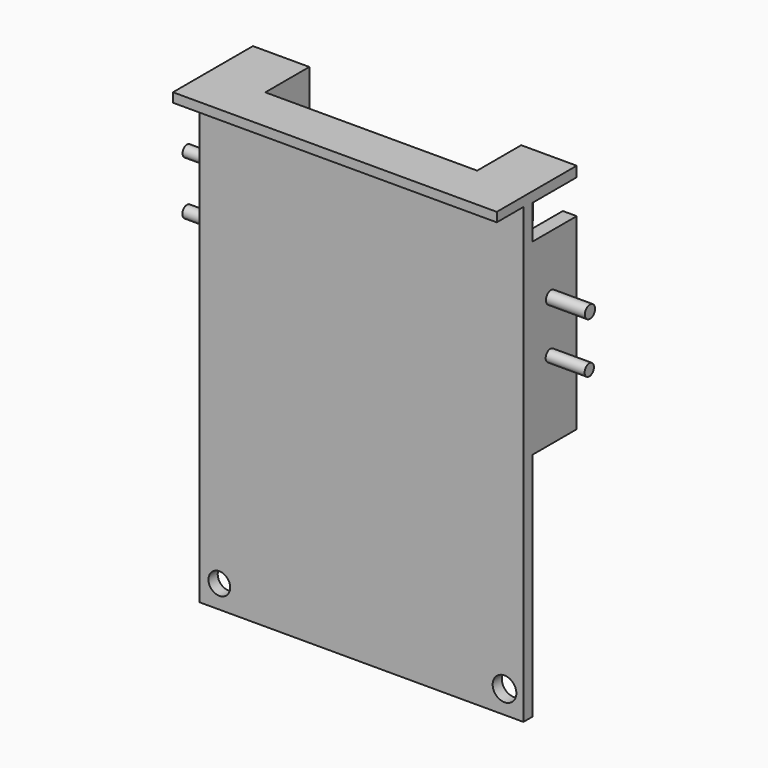
from build123d import *

# Parameters (mm, degrees)
F0_W     = 88.9
F0_H     = 127
F0_R     = 2.9848451786
F0_R_2   = 3.2536679358
F1_DEPTH = 3.175
F2_W     = 88.9
F2_H     = 2.54
F3_DEPTH = 9.14618
F4_W     = 3.1831779712
F4_H     = 14.4224017859
F4_W_2   = 3.8154479831
F4_H_2   = 51.5085849911
F4_W_3   = 2.9760506004
F4_H_3   = 14.1934752464
F4_W_4   = 3.5865214437
F4_H_4   = 51.7375124618
F5_DEPTH = 15.11912
F6_R     = 1.7434569234
F6_R_2   = 1.6024885699
F7_DEPTH = 10.69614
F8_R     = 1.5356896605
F8_R_2   = 1.6187597598
F9_DEPTH = 12.03988


with BuildPart() as f1:
    # F0 (on Front) → F1 (new body)
    with BuildSketch(Plane.XZ):
        with Locations((-0.1144651324, -7.7015060779)):
            Rectangle(F0_W, F0_H)
        with Locations((-39.1465239227, -64.9008154869)):
            Circle(F0_R, mode=Mode.SUBTRACT)
        with Locations((39.1465201974, -64.9008154869)):
            Circle(F0_R_2, mode=Mode.SUBTRACT)
    extrude(amount=F1_DEPTH)

    # F2 (on face) → F3 (join)
    with BuildSketch(Plane.XZ.offset(3.175)):
        with Locations((-0.1144651324, 54.5284939221)):
            Rectangle(F2_W, F2_H)
    extrude(amount=F3_DEPTH)

    # F4 (on face) → F5 (join)
    with BuildSketch(Plane(origin=(0, 0, 0), x_dir=(-1, 0, 0), z_dir=(0, 1, 0))):
        Polygon((-29.0955348676, 55.4166970754), (-29.0955348676, 55.7984939221), (-44.3355348676, 55.7984939221), (-44.3355348676, 55.4166970754), (-44.3355348676, 52.99660936), (-32.2787128389, 52.99660936), (-29.0955348676, 52.99660936), align=None)
        with Locations((-30.6871238533, 45.7854084671)):
            Rectangle(F4_W, F4_H)
        with Locations((-42.4278108761, 17.8563101217)):
            Rectangle(F4_W_2, F4_H_2)
        Polygon((44.5644651324, 55.7984939221), (29.0737356991, 55.7984939221), (29.0737356991, 53.2255358994), (32.0497862995, 53.2255358994), (40.7490134239, 53.2255358994), (44.5644651324, 53.2255358994), align=None)
        with Locations((30.5617609993, 46.1287982762)):
            Rectangle(F4_W_3, F4_H_3)
        with Locations((42.7712044105, 17.7418463863)):
            Rectangle(F4_W_4, F4_H_4)
    extrude(amount=F5_DEPTH)

    # F6 (on face) → F7 (join)
    with BuildSketch(Plane.YZ.offset(44.3355348676)):
        with Locations((6.2954924069, 27.5857094675)):
            Circle(F6_R)
        with Locations((6.0665672645, 13.6211588979)):
            Circle(F6_R_2)
    extrude(amount=F7_DEPTH)

    # F8 (on face) → F9 (join)
    with BuildSketch(Plane(origin=(-44.5644651324, 0, 0), x_dir=(0, -1, 0), z_dir=(-1, 0, 0))):
        with Locations((-7.554592099, 29.6460520476)):
            Circle(F8_R)
        with Locations((-7.554592099, 14.9947218597)):
            Circle(F8_R_2)
    extrude(amount=F9_DEPTH)


solid = f1.part
